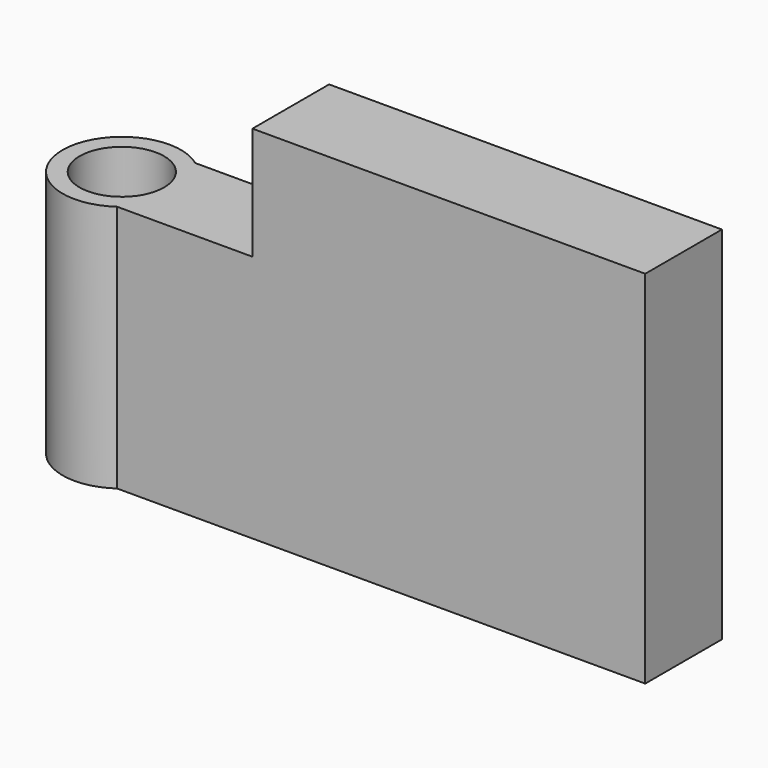
from build123d import *

# Parameters (mm, degrees)
F0_R     = 1.875
F1_DEPTH = 11
F2_W     = 17.4188611699
F2_H     = 4.25
F3_DEPTH = 5


# Not quite as in the source:
# - a feature names something its author has since deleted; it is built from what else it names


with BuildPart() as f1:
    # F0 (on Top) → F1 (new body)
    with BuildSketch(Plane.XY):
        with BuildLine():
            ThreePointArc((1.5092688833, -2.1477272727), (2.3294265194, -1.2101227585), (2.625, 0))
            ThreePointArc((2.625, 0), (2.347022952, 1.1756310061), (1.5719651333, 2.1022727273))
            ThreePointArc((1.5719651333, 2.1022727273), (-2.6247144161, 0.0387199415), (1.5092688833, -2.1477272727))
        make_face()
        Circle(F0_R, mode=Mode.SUBTRACT)
        with BuildLine():
            ThreePointArc((1.5719651333, 2.1022727273), (2.347022952, 1.1756310061), (2.625, 0))
            ThreePointArc((2.625, 0), (2.3294265194, -1.2101227585), (1.5092688833, -2.1477272727))
            Line((1.5092688833, -2.1477272727), (24.9281300532, -2.1477272727))
            Line((24.9281300532, -2.1477272727), (24.9281300532, 2.1022727273))
            Line((24.9281300532, 2.1022727273), (1.5719651333, 2.1022727273))
        make_face()
    extrude(amount=F1_DEPTH)

    # F2 (on face) → F3 (join)
    with BuildSketch(Plane.XY.offset(11)):
        with Locations((16.2186994682, -0.0227272727)):
            Rectangle(F2_W, F2_H)
    extrude(amount=F3_DEPTH)


solid = f1.part
